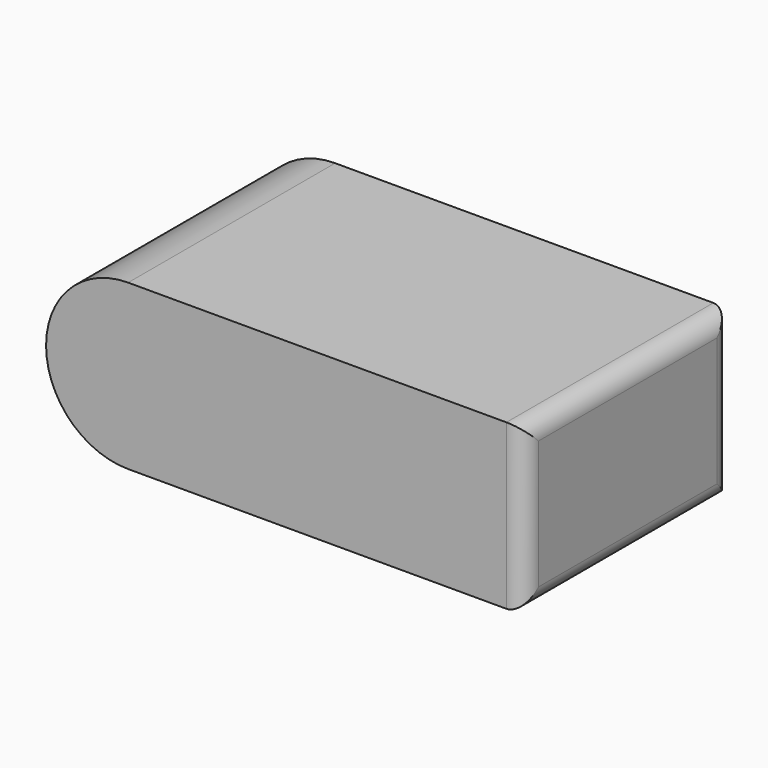
from build123d import *

# Parameters (mm, degrees)
F0_W     = 53.6
F0_H     = 29
F1_DEPTH = 18.4
F2_R     = 9.19999
F3_R     = 2


# Not quite as in the source:
# - a fillet or chamfer is up to 0.001 mm smaller than in the source, because OpenCascade refuses the exact size


with BuildPart() as f1:
    # F0 (on Top) → F1 (new body)
    with BuildSketch(Plane.XY):
        Rectangle(F0_W, F0_H)
    extrude(amount=F1_DEPTH)

    # F2 (radius 9.2 in the source; OpenCascade refuses exactly that, so slightly less here)
    f2_edges = [f1.edges().sort_by_distance(p)[0] for p in [
        (-26.8, 0, 18.4),
        (-26.8, 0, 0),
    ]]
    fillet(f2_edges, radius=F2_R)

    # F3
    f3_edges = [f1.edges().sort_by_distance(p)[0] for p in [
        (26.8, -14.5, 9.2),
        (26.8, 14.5, 9.2),
        (26.8, 0, 0),
        (26.8, 0, 18.4),
    ]]
    fillet(f3_edges, radius=F3_R)


solid = f1.part
